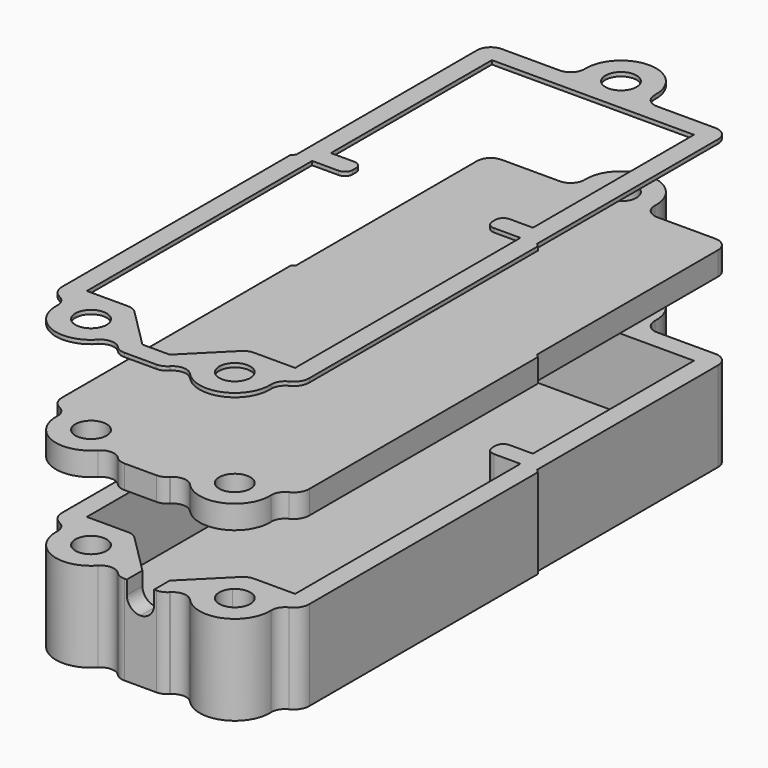
from build123d import *

# Parameters (mm, degrees)
F1_DEPTH  = 2.5
F0_R      = 2
F2_DEPTH  = 11.5
F0_W      = 3.5
F0_H      = 2.5
F3_DEPTH  = 8
F4_R      = 1.74999
F5_SIZE   = 0.35
F6_R      = 2
F8_R      = 2
F9_DEPTH  = 3
F10_R     = 1
F12_R     = 2
F13_DEPTH = 0.5


# Not quite as in the source:
# - a fillet or chamfer is up to 0.001 mm smaller than in the source, because OpenCascade refuses the exact size


with BuildPart() as f1:
    # F0 (on Top) → F1 (new body)
    with BuildSketch(Plane.XY):
        Polygon((8.95, -12.9), (12.95, -12.9), (12.95, 12.9), (-12.95, 12.9), (-12.95, -12.9), (-8.95, -12.9), (-8.95, -15.4), (-13.35, -15.4), (-13.35, -51.5), (-7.35, -51.5), (-1.75, -57.1), (1.75, -57.1), (7.35, -51.5), (13.35, -51.5), (13.35, -15.4), (8.95, -15.4), align=None)
    extrude(amount=F1_DEPTH)

    # F0 (on Top) → F2 (join)
    with BuildSketch(Plane.XY):
        with BuildLine():
            Line((12.95, 12.9), (12.95, -12.9))
            Line((12.95, -12.9), (8.95, -12.9))
            Line((8.95, -12.9), (8.95, -15.4))
            Line((8.95, -15.4), (13.35, -15.4))
            Line((13.35, -15.4), (15.45, -15.4))
            Line((15.45, -15.4), (15.45, 15.4))
            Line((15.45, 15.4), (4.0311288741, 15.4))
            ThreePointArc((4.0311288741, 15.4), (0, 21.9), (-4.0311288741, 15.4))
            Line((-4.0311288741, 15.4), (-15.45, 15.4))
            Line((-15.45, 15.4), (-15.45, -15.4))
            Line((-15.45, -15.4), (-13.35, -15.4))
            Line((-13.35, -15.4), (-8.95, -15.4))
            Line((-8.95, -15.4), (-8.95, -12.9))
            Line((-8.95, -12.9), (-12.95, -12.9))
            Line((-12.95, -12.9), (-12.95, 12.9))
            Line((-12.95, 12.9), (12.95, 12.9))
        make_face()
        with Locations((0, 17.4)):
            Circle(F0_R, mode=Mode.SUBTRACT)
        with BuildLine():
            Line((-13.35, -51.5), (-13.35, -15.4))
            Line((-13.35, -15.4), (-15.45, -15.4))
            Line((-15.45, -15.4), (-15.85, -15.4))
            Line((-15.85, -15.4), (-15.85, -54))
            Line((-15.85, -54), (-13.2450899048, -54))
            ThreePointArc((-13.2450899048, -54), (-10.9360364763, -60.1574578963), (-4.9493089056, -57.4362250004))
            Line((-4.9493089056, -57.4362250004), (-2.7855339059, -59.6))
            Line((-2.7855339059, -59.6), (-1.75, -59.6))
            Line((-1.75, -59.6), (-1.75, -57.1))
            Line((-1.75, -57.1), (-7.35, -51.5))
            Line((-7.35, -51.5), (-13.35, -51.5))
        make_face()
        with Locations((-9.2139610307, -56)):
            Circle(F0_R, mode=Mode.SUBTRACT)
        with BuildLine():
            Line((15.45, -15.4), (13.35, -15.4))
            Line((13.35, -15.4), (13.35, -51.5))
            Line((13.35, -51.5), (7.35, -51.5))
            Line((7.35, -51.5), (1.75, -57.1))
            Line((1.75, -57.1), (1.75, -59.6))
            Line((1.75, -59.6), (2.7855339059, -59.6))
            Line((2.7855339059, -59.6), (4.9493089056, -57.4362250004))
            ThreePointArc((4.9493089056, -57.4362250004), (10.9360364763, -60.1574578963), (13.2450899048, -54))
            Line((13.2450899048, -54), (15.85, -54))
            Line((15.85, -54), (15.85, -15.4))
            Line((15.85, -15.4), (15.45, -15.4))
        make_face()
        with BuildLine():
            ThreePointArc((11.2139610307, -56), (8.4485941659, -57.847759065), (7.7997474683, -54.5857864376))
            ThreePointArc((7.7997474683, -54.5857864376), (9.9793278954, -54.152240935), (11.2139610307, -56))
        make_face(mode=Mode.SUBTRACT)
    extrude(amount=F2_DEPTH)

    # F0 (on Top) → F3 (join)
    with BuildSketch(Plane.XY):
        with Locations((0, -58.35)):
            Rectangle(F0_W, F0_H)
    extrude(amount=F3_DEPTH)

    # F4 (radius 1.75 in the source; OpenCascade refuses exactly that, so slightly less here)
    f4_edges = [f1.edges().sort_by_distance(p)[0] for p in [
        (-1.75, -58.35, 8),
        (1.75, -58.35, 8),
        (-13.24509, -54, 5.75),
        (-4.949309, -57.436225, 5.75),
        (4.949309, -57.436225, 5.75),
        (13.24509, -54, 5.75),
        (2.785534, -59.6, 5.75),
        (-2.785534, -59.6, 5.75),
        (-4.031129, 15.4, 5.75),
        (4.031129, 15.4, 5.75),
        (15.45, 15.4, 5.75),
        (-15.45, 15.4, 5.75),
        (7.35, -51.5, 7),
        (-7.35, -51.5, 7),
    ]]
    fillet(f4_edges, radius=F4_R)

    # F5
    f5_edges = [f1.edges().sort_by_distance(p)[0] for p in [
        (15.85, -15.4, 5.75),
        (-15.85, -15.4, 5.75),
    ]]
    chamfer(f5_edges, length=F5_SIZE)

    # F6
    f6_edges = [f1.edges().sort_by_distance(p)[0] for p in [
        (-15.85, -54, 5.75),
        (15.85, -54, 5.75),
    ]]
    fillet(f6_edges, radius=F6_R)

    # F10
    f10_edges = [f1.edges().sort_by_distance(p)[0] for p in [
        (-8.95, -15.4, 7),
        (8.95, -15.4, 7),
        (-8.95, -12.9, 7),
        (8.95, -12.9, 7),
    ]]
    fillet(f10_edges, radius=F10_R)


with BuildPart() as f9:
    # F8 (on offset) → F9 (new body)
    with BuildSketch(Plane.XY.offset(21.5)):
        with BuildLine():
            Line((-15.45, -15.35), (-15.85, -15.75))
            Line((-15.85, -15.75), (-15.85, -52.3627074465))
            ThreePointArc((-15.85, -52.3627074465), (-15.5405950083, -53.4312992853), (-14.7081114822, -54.1692634751))
            ThreePointArc((-14.7081114822, -54.1692634751), (-13.9612802991, -54.8447605721), (-13.7103595895, -55.82))
            ThreePointArc((-13.7103595895, -55.82), (-10.9360364763, -60.1574578963), (-5.9072478982, -59.0521546913))
            ThreePointArc((-5.9072478982, -59.0521546913), (-4.6563109071, -58.489453913), (-3.3838670351, -59.0016668708))
            Line((-3.3838670351, -59.0016668708), (-3.2980970389, -59.0874368671))
            ThreePointArc((-3.2980970389, -59.0874368671), (-2.7303561784, -59.4667891819), (-2.0606601718, -59.6))
            Line((-2.0606601718, -59.6), (-1.75, -59.6))
            Line((-1.75, -59.6), (1.75, -59.6))
            Line((1.75, -59.6), (2.0606601718, -59.6))
            ThreePointArc((2.0606601718, -59.6), (2.7303561784, -59.4667891819), (3.2980970389, -59.0874368671))
            Line((3.2980970389, -59.0874368671), (3.3838670351, -59.0016668708))
            ThreePointArc((3.3838670351, -59.0016668708), (4.6563109071, -58.489453913), (5.9072478982, -59.0521546913))
            ThreePointArc((5.9072478982, -59.0521546913), (10.9360364763, -60.1574578963), (13.7103595895, -55.82))
            ThreePointArc((13.7103595895, -55.82), (13.9612802991, -54.8447605721), (14.7081114822, -54.1692634751))
            ThreePointArc((14.7081114822, -54.1692634751), (15.5405950083, -53.4312992853), (15.85, -52.3627074465))
            Line((15.85, -52.3627074465), (15.85, -15.75))
            Line((15.85, -15.75), (15.45, -15.35))
            Line((15.45, -15.35), (15.45, 13.65))
            ThreePointArc((15.45, 13.65), (14.9374368671, 14.8874368671), (13.7, 15.4))
            Line((13.7, 15.4), (6.2449979984, 15.4))
            ThreePointArc((6.2449979984, 15.4), (4.983055052, 15.9375644347), (4.4963985588, 17.22))
            ThreePointArc((4.4963985588, 17.22), (0, 21.9), (-4.4963985588, 17.22))
            ThreePointArc((-4.4963985588, 17.22), (-4.983055052, 15.9375644347), (-6.2449979984, 15.4))
            Line((-6.2449979984, 15.4), (-13.7, 15.4))
            ThreePointArc((-13.7, 15.4), (-14.9374368671, 14.8874368671), (-15.45, 13.65))
            Line((-15.45, 13.65), (-15.45, -15.35))
        make_face()
        with Locations((-9.2139610307, -56)):
            Circle(F8_R, mode=Mode.SUBTRACT)
        with Locations((9.2139610307, -56)):
            Circle(F8_R, mode=Mode.SUBTRACT)
        with Locations((0, 17.4)):
            Circle(F8_R, mode=Mode.SUBTRACT)
    extrude(amount=F9_DEPTH)


with BuildPart() as f13:
    # F12 (on offset) → F13 (new body)
    with BuildSketch(Plane.XY.offset(36.5)):
        with BuildLine():
            Line((-1.75, -59.6), (1.75, -59.6))
            Line((1.75, -59.6), (2.0606601718, -59.6))
            ThreePointArc((2.0606601718, -59.6), (2.7303561784, -59.4667891819), (3.2980970389, -59.0874368671))
            Line((3.2980970389, -59.0874368671), (3.3838670351, -59.0016668708))
            ThreePointArc((3.3838670351, -59.0016668708), (4.6563109071, -58.489453913), (5.9072478982, -59.0521546913))
            ThreePointArc((5.9072478982, -59.0521546913), (10.9360364763, -60.1574578963), (13.7103595895, -55.82))
            ThreePointArc((13.7103595895, -55.82), (13.9612802991, -54.8447605721), (14.7081114822, -54.1692634751))
            ThreePointArc((14.7081114822, -54.1692634751), (15.5405950083, -53.4312992853), (15.85, -52.3627074465))
            Line((15.85, -52.3627074465), (15.85, -15.75))
            Line((15.85, -15.75), (15.45, -15.35))
            Line((15.45, -15.35), (15.45, 13.65))
            ThreePointArc((15.45, 13.65), (14.9374368671, 14.8874368671), (13.7, 15.4))
            Line((13.7, 15.4), (6.2449979984, 15.4))
            ThreePointArc((6.2449979984, 15.4), (4.983055052, 15.9375644347), (4.4963985588, 17.22))
            ThreePointArc((4.4963985588, 17.22), (0, 21.9), (-4.4963985588, 17.22))
            ThreePointArc((-4.4963985588, 17.22), (-4.983055052, 15.9375644347), (-6.2449979984, 15.4))
            Line((-6.2449979984, 15.4), (-13.7, 15.4))
            ThreePointArc((-13.7, 15.4), (-14.9374368671, 14.8874368671), (-15.45, 13.65))
            Line((-15.45, 13.65), (-15.45, -15.35))
            Line((-15.45, -15.35), (-15.85, -15.75))
            Line((-15.85, -15.75), (-15.85, -52.3627074465))
            ThreePointArc((-15.85, -52.3627074465), (-15.5405950083, -53.4312992853), (-14.7081114822, -54.1692634751))
            ThreePointArc((-14.7081114822, -54.1692634751), (-13.9612802991, -54.8447605721), (-13.7103595895, -55.82))
            ThreePointArc((-13.7103595895, -55.82), (-10.9360364763, -60.1574578963), (-5.9072478982, -59.0521546913))
            ThreePointArc((-5.9072478982, -59.0521546913), (-4.6563109071, -58.489453913), (-3.3838670351, -59.0016668708))
            Line((-3.3838670351, -59.0016668708), (-3.2980970389, -59.0874368671))
            ThreePointArc((-3.2980970389, -59.0874368671), (-2.7303561784, -59.4667891819), (-2.0606601718, -59.6))
            Line((-2.0606601718, -59.6), (-1.75, -59.6))
        make_face()
        with Locations((-9.2139610307, -56)):
            Circle(F12_R, mode=Mode.SUBTRACT)
        with BuildLine():
            Line((-13.35, -51.5), (-13.35, -15.4))
            Line((-13.35, -15.4), (-9.95, -15.4))
            ThreePointArc((-9.95, -15.4), (-9.2428932188, -15.1071067812), (-8.95, -14.4))
            Line((-8.95, -14.4), (-8.95, -13.9))
            ThreePointArc((-8.95, -13.9), (-9.2428932188, -13.1928932188), (-9.95, -12.9))
            Line((-9.95, -12.9), (-12.95, -12.9))
            Line((-12.95, -12.9), (-12.95, 12.9))
            Line((-12.95, 12.9), (12.95, 12.9))
            Line((12.95, 12.9), (12.95, -12.9))
            Line((12.95, -12.9), (9.95, -12.9))
            ThreePointArc((9.95, -12.9), (9.2428932188, -13.1928932188), (8.95, -13.9))
            Line((8.95, -13.9), (8.95, -14.4))
            ThreePointArc((8.95, -14.4), (9.2428932188, -15.1071067812), (9.95, -15.4))
            Line((9.95, -15.4), (13.35, -15.4))
            Line((13.35, -15.4), (13.35, -51.5))
            Line((13.35, -51.5), (8.0748737342, -51.5))
            ThreePointArc((8.0748737342, -51.5), (7.4051777275, -51.6332108181), (6.8374368671, -52.0125631329))
            Line((6.8374368671, -52.0125631329), (1.75, -57.1))
            Line((1.75, -57.1), (-1.75, -57.1))
            Line((-1.75, -57.1), (-6.8374368671, -52.0125631329))
            ThreePointArc((-6.8374368671, -52.0125631329), (-7.4051777275, -51.6332108181), (-8.0748737342, -51.5))
            Line((-8.0748737342, -51.5), (-13.35, -51.5))
        make_face(mode=Mode.SUBTRACT)
        with Locations((9.2139610307, -56)):
            Circle(F12_R, mode=Mode.SUBTRACT)
        with Locations((0, 17.4)):
            Circle(F12_R, mode=Mode.SUBTRACT)
    extrude(amount=F13_DEPTH)


solid = Compound([f1.part, f9.part, f13.part])
